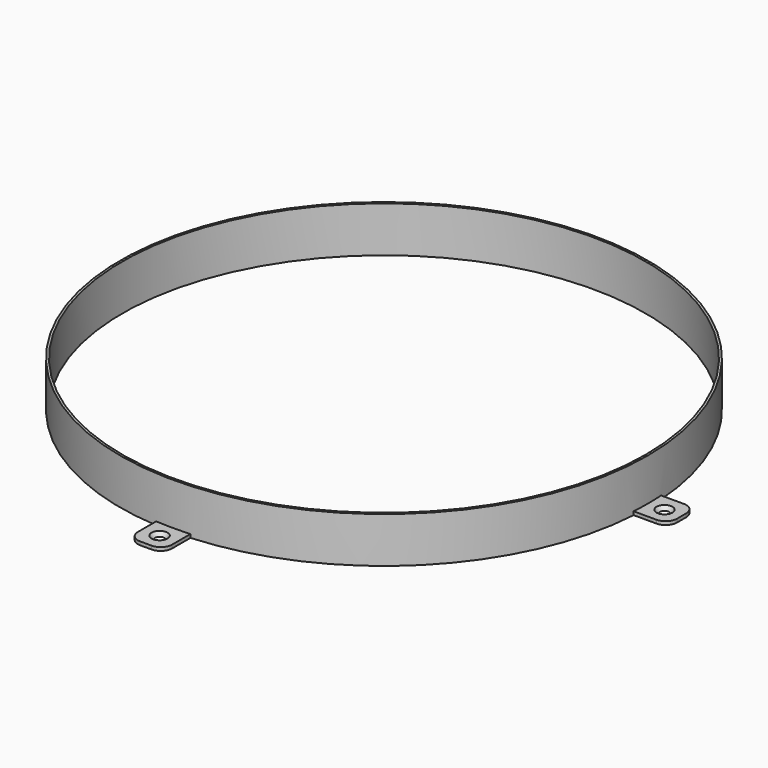
from build123d import *

# Parameters (mm, degrees)
F0_R     = 231
F0_R_2   = 229
F1_DEPTH = 40
F2_W     = 30
F2_H     = 30
F3_DEPTH = 3
F4_R     = 4
F5_DEPTH = 25
F6_R     = 10
F8_COUNT = 4
F9_SIZE  = 2.99999


# Not quite as in the source:
# - a fillet or chamfer is up to 0.001 mm smaller than in the source, because OpenCascade refuses the exact size


with BuildPart() as f1:
    # F0 (on Top) → F1 (new body)
    with BuildSketch(Plane.XY):
        Circle(F0_R)
        Circle(F0_R_2, mode=Mode.SUBTRACT)
    extrude(amount=F1_DEPTH)

    # F2 (on face) → F3 (join)
    with BuildSketch(Plane(origin=(0, 0, 0), x_dir=(1, 0, 0), z_dir=(0, 0, -1))):
        with Locations((0, -245.5124725476)):
            Rectangle(F2_W, F2_H)
    extrude(amount=-F3_DEPTH)

    # F4 (on face) → F5 (cut)
    with BuildSketch(Plane(origin=(0, 0, 0), x_dir=(1, 0, 0), z_dir=(0, 0, -1))):
        with Locations((0, -245.5124725476)):
            Circle(F4_R)
    extrude(amount=-F5_DEPTH, mode=Mode.SUBTRACT)

    # F6
    f6_edges = [f1.edges().sort_by_distance(p)[0] for p in [
        (-15, 260.512473, 1.5),
        (15, 260.512473, 1.5),
    ]]
    fillet(f6_edges, radius=F6_R)

    # F8: F1 ×4 about axis
    f8_axis = Axis((0, 0, -51.1162020266), (0, 0, -1))


with BuildPart() as f1_1:
    add(f1.part)
    for i in range(1, F8_COUNT):
        add(f1.part.rotate(f8_axis, i * 360 / F8_COUNT))

    # F9 (size 3 in the source; OpenCascade refuses exactly that, so slightly less here)
    f9_edges = [f1_1.edges().sort_by_distance(p)[0] for p in [
        (-245.512473, -4, 3),
        (-4, 245.512473, 3),
        (245.512473, 4, 3),
        (4, -245.512473, 3),
    ]]
    chamfer(f9_edges, length=F9_SIZE)


solid = f1_1.part
